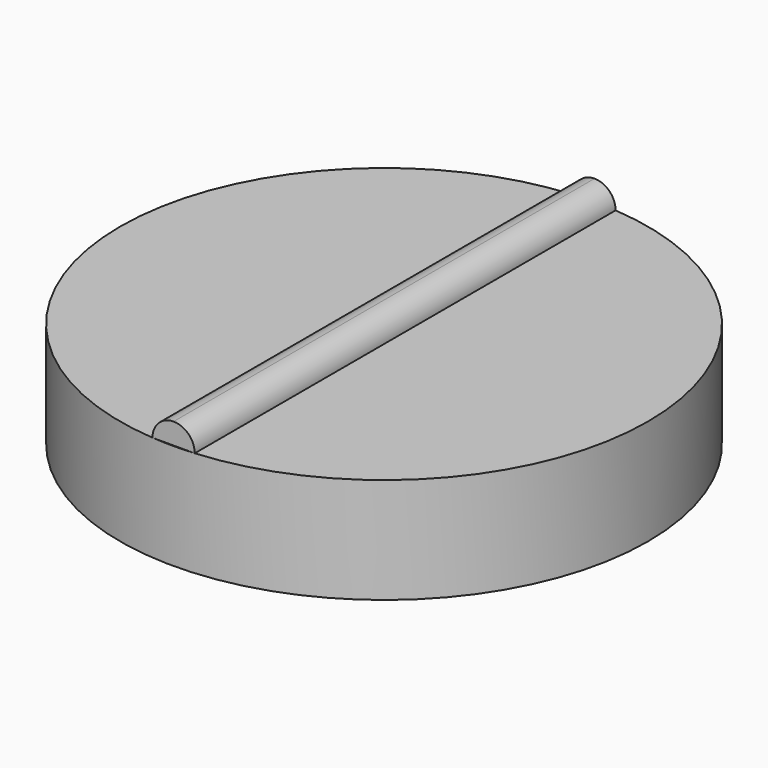
from build123d import *

# Parameters (mm, degrees)
F0_R     = 12.5
F1_DEPTH = 5
F2_W     = 2
F2_H     = 24.9198715888
F3_DEPTH = 1
F4_R     = 0.99999


# Not quite as in the source:
# - a fillet or chamfer is up to 0.001 mm smaller than in the source, because OpenCascade refuses the exact size


with BuildPart() as f1:
    # F0 (on Top) → F1 (new body)
    with BuildSketch(Plane.XY):
        Circle(F0_R)
    extrude(amount=F1_DEPTH)

    # F2 (on face) → F3 (join)
    with BuildSketch(Plane.XY.offset(5)):
        Rectangle(F2_W, F2_H)
    extrude(amount=F3_DEPTH)

    # F4 (radius 1 in the source; OpenCascade refuses exactly that, so slightly less here)
    f4_edges = [f1.edges().sort_by_distance(p)[0] for p in [
        (1, 0, 6),
        (-1, 0, 6),
    ]]
    fillet(f4_edges, radius=F4_R)


solid = f1.part
